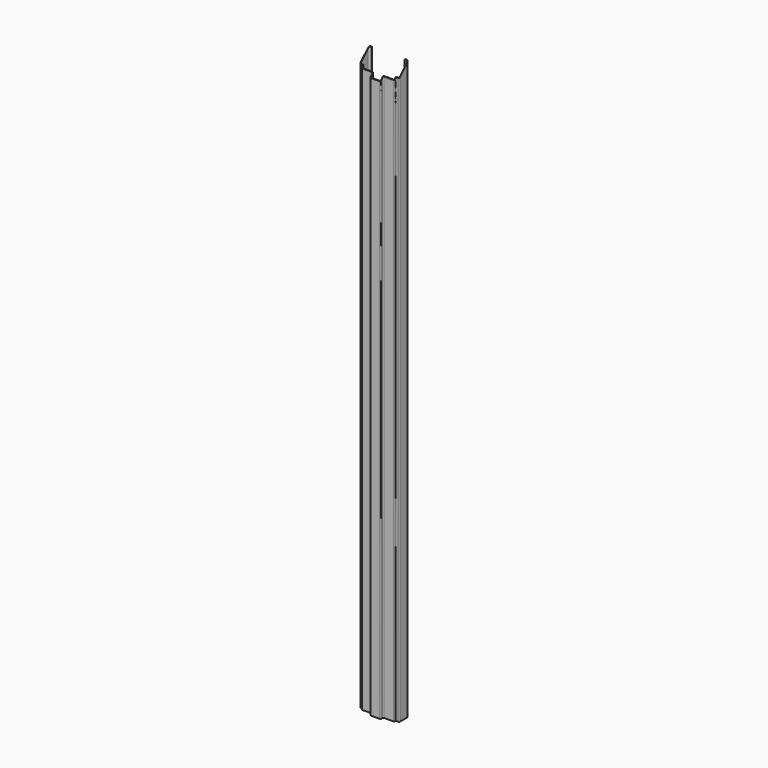
from build123d import *

# Parameters (mm, degrees)
F1_DEPTH     = 2070
F2_T1_DEPTH  = 2070
F2_T3_DEPTH  = 2070
F2_T5_DEPTH  = 2070
F2_T7_DEPTH  = 2070
F2_T9_DEPTH  = 2070
F2_T11_DEPTH = 2070
F2_T13_DEPTH = 2070
F2_T15_DEPTH = 2070
F2_T17_DEPTH = 2070
F2_T19_DEPTH = 2070
F2_T21_DEPTH = 2070
F2_T23_DEPTH = 2070
F2_T25_DEPTH = 2085
F2_T27_DEPTH = 2085
F2_T29_DEPTH = 2085
F2_T31_DEPTH = 2085
F2_T33_DEPTH = 2085
F2_T35_DEPTH = 2085
F2_T37_DEPTH = 2085
F2_T39_DEPTH = 2085
F2_T41_DEPTH = 2085
F2_T43_DEPTH = 2085
F2_T45_DEPTH = 2085
F2_T47_DEPTH = 2085
F3_R         = 5
F6_DEPTH     = 166


# Not quite as in the source:
# - a fillet or chamfer that OpenCascade refuses, or shapes differently, is made with other operations: its cross-section is extruded or revolved along the edge and cut away or added


with BuildPart() as f1:
    # F0 (on Top) → F1 (new body)
    with BuildSketch(Plane.XY):
        Polygon((-18.5, 0), (0, 0), (18.5, 0), (18.5, 12), (58.5, 12), (58.5, 19), (70.5, 19), (70.5, 60), (58.5, 60), (58.5, 57), (59.5, 57), (59.5, 59), (69.5, 59), (69.5, 20), (57.5, 20), (57.5, 13), (17.5, 13), (17.5, 1), (0, 1), (-17.5, 1), (-17.5, 13), (-57.5, 13), (-57.5, 20), (-69.5, 20), (-69.5, 59), (-59.5, 59), (-59.5, 57), (-58.5, 57), (-58.5, 60), (-70.5, 60), (-70.5, 19), (-58.5, 19), (-58.5, 12), (-18.5, 12), align=None)
    extrude(amount=F1_DEPTH)

    # F2: fillet of radius 3 on 24 edges, made by hand

    # F2_s2 → F2_t1 (join)
    with BuildSketch(Plane.XY):
        with BuildLine():
            add(Edge.make_bspline(
                [(-21.5, 12), (-18.5, 12), (-18.5, 9)],
                knots=[0, 0, 0, 1, 1, 1], degree=2, weights=[1, 1, 1]))
            Line((-18.5, 9), (-18.5, 12))
            Line((-18.5, 12), (-21.5, 12))
        make_face()
    extrude(amount=F2_T1_DEPTH)

    # F2_s4 → F2_t3 (join)
    with BuildSketch(Plane.XY):
        with BuildLine():
            add(Edge.make_bspline(
                [(-61.5, 19), (-58.5, 19), (-58.5, 16)],
                knots=[0, 0, 0, 1, 1, 1], degree=2, weights=[1, 1, 1]))
            Line((-58.5, 16), (-58.5, 19))
            Line((-58.5, 19), (-61.5, 19))
        make_face()
    extrude(amount=F2_T3_DEPTH)

    # F2_s6 → F2_t5 (join)
    with BuildSketch(Plane.XY):
        with BuildLine():
            add(Edge.make_bspline(
                [(-62.3284271247, 59), (-60.2071067812, 59), (-59.5, 57)],
                knots=[0, 0, 0, 1, 1, 1], degree=2, weights=[1, 1, 1]))
            Line((-59.5, 57), (-59.5, 59))
            Line((-59.5, 59), (-62.3284271247, 59))
        make_face()
    extrude(amount=F2_T5_DEPTH)

    # F2_s8 → F2_t7 (join)
    with BuildSketch(Plane.XY):
        with BuildLine():
            add(Edge.make_bspline(
                [(-66.5, 20), (-69.5, 20), (-69.5, 23)],
                knots=[0, 0, 0, 1, 1, 1], degree=2, weights=[1, 1, 1]))
            Line((-69.5, 23), (-69.5, 20))
            Line((-69.5, 20), (-66.5, 20))
        make_face()
    extrude(amount=F2_T7_DEPTH)

    # F2_s10 → F2_t9 (join)
    with BuildSketch(Plane.XY):
        with BuildLine():
            add(Edge.make_bspline(
                [(-54.5, 13), (-57.5, 13), (-57.5, 16)],
                knots=[0, 0, 0, 1, 1, 1], degree=2, weights=[1, 1, 1]))
            Line((-57.5, 16), (-57.5, 13))
            Line((-57.5, 13), (-54.5, 13))
        make_face()
    extrude(amount=F2_T9_DEPTH)

    # F2_s12 → F2_t11 (join)
    with BuildSketch(Plane.XY):
        with BuildLine():
            add(Edge.make_bspline(
                [(-14.5, 1), (-17.5, 1), (-17.5, 4)],
                knots=[0, 0, 0, 1, 1, 1], degree=2, weights=[1, 1, 1]))
            Line((-17.5, 4), (-17.5, 1))
            Line((-17.5, 1), (-14.5, 1))
        make_face()
    extrude(amount=F2_T11_DEPTH)

    # F2_s14 → F2_t13 (join)
    with BuildSketch(Plane.XY):
        with BuildLine():
            add(Edge.make_bspline(
                [(17.5, 4), (17.5, 1), (14.5, 1)],
                knots=[0, 0, 0, 1, 1, 1], degree=2, weights=[1, 1, 1]))
            Line((14.5, 1), (17.5, 1))
            Line((17.5, 1), (17.5, 4))
        make_face()
    extrude(amount=F2_T13_DEPTH)

    # F2_s16 → F2_t15 (join)
    with BuildSketch(Plane.XY):
        with BuildLine():
            add(Edge.make_bspline(
                [(57.5, 16), (57.5, 13), (54.5, 13)],
                knots=[0, 0, 0, 1, 1, 1], degree=2, weights=[1, 1, 1]))
            Line((54.5, 13), (57.5, 13))
            Line((57.5, 13), (57.5, 16))
        make_face()
    extrude(amount=F2_T15_DEPTH)

    # F2_s18 → F2_t17 (join)
    with BuildSketch(Plane.XY):
        with BuildLine():
            add(Edge.make_bspline(
                [(69.5, 23), (69.5, 20), (66.5, 20)],
                knots=[0, 0, 0, 1, 1, 1], degree=2, weights=[1, 1, 1]))
            Line((66.5, 20), (69.5, 20))
            Line((69.5, 20), (69.5, 23))
        make_face()
    extrude(amount=F2_T17_DEPTH)

    # F2_s20 → F2_t19 (join)
    with BuildSketch(Plane.XY):
        with BuildLine():
            add(Edge.make_bspline(
                [(59.5, 57), (60.2071067812, 59), (62.3284271247, 59)],
                knots=[0, 0, 0, 1, 1, 1], degree=2, weights=[1, 1, 1]))
            Line((62.3284271247, 59), (59.5, 59))
            Line((59.5, 59), (59.5, 57))
        make_face()
    extrude(amount=F2_T19_DEPTH)

    # F2_s22 → F2_t21 (join)
    with BuildSketch(Plane.XY):
        with BuildLine():
            add(Edge.make_bspline(
                [(58.5, 16), (58.5, 19), (61.5, 19)],
                knots=[0, 0, 0, 1, 1, 1], degree=2, weights=[1, 1, 1]))
            Line((61.5, 19), (58.5, 19))
            Line((58.5, 19), (58.5, 16))
        make_face()
    extrude(amount=F2_T21_DEPTH)

    # F2_s24 → F2_t23 (join)
    with BuildSketch(Plane.XY):
        with BuildLine():
            add(Edge.make_bspline(
                [(18.5, 9), (18.5, 12), (21.5, 12)],
                knots=[0, 0, 0, 1, 1, 1], degree=2, weights=[1, 1, 1]))
            Line((21.5, 12), (18.5, 12))
            Line((18.5, 12), (18.5, 9))
        make_face()
    extrude(amount=F2_T23_DEPTH)

    # F2_s26 → F2_t25 (cut)
    with BuildSketch(Plane.XY.offset(-7.5)):
        with BuildLine():
            add(Edge.make_bspline(
                [(-15.5, 0), (-18.5, 0), (-18.5, 3)],
                knots=[0, 0, 0, 1, 1, 1], degree=2, weights=[1, 1, 1]))
            Line((-18.5, 3), (-18.5, 0))
            Line((-18.5, 0), (-15.5, 0))
        make_face()
    extrude(amount=F2_T25_DEPTH, mode=Mode.SUBTRACT)

    # F2_s28 → F2_t27 (cut)
    with BuildSketch(Plane.XY.offset(-7.5)):
        with BuildLine():
            add(Edge.make_bspline(
                [(15.5, 0), (18.5, 0), (18.5, 3)],
                knots=[0, 0, 0, 1, 1, 1], degree=2, weights=[1, 1, 1]))
            Line((18.5, 3), (18.5, 0))
            Line((18.5, 0), (15.5, 0))
        make_face()
    extrude(amount=F2_T27_DEPTH, mode=Mode.SUBTRACT)

    # F2_s30 → F2_t29 (cut)
    with BuildSketch(Plane.XY.offset(-7.5)):
        with BuildLine():
            add(Edge.make_bspline(
                [(-55.5, 12), (-58.5, 12), (-58.5, 15)],
                knots=[0, 0, 0, 1, 1, 1], degree=2, weights=[1, 1, 1]))
            Line((-58.5, 15), (-58.5, 12))
            Line((-58.5, 12), (-55.5, 12))
        make_face()
    extrude(amount=F2_T29_DEPTH, mode=Mode.SUBTRACT)

    # F2_s32 → F2_t31 (cut)
    with BuildSketch(Plane.XY.offset(-7.5)):
        with BuildLine():
            add(Edge.make_bspline(
                [(-67.5, 19), (-70.5, 19), (-70.5, 22)],
                knots=[0, 0, 0, 1, 1, 1], degree=2, weights=[1, 1, 1]))
            Line((-70.5, 22), (-70.5, 19))
            Line((-70.5, 19), (-67.5, 19))
        make_face()
    extrude(amount=F2_T31_DEPTH, mode=Mode.SUBTRACT)

    # F2_s34 → F2_t33 (cut)
    with BuildSketch(Plane.XY.offset(-7.5)):
        with BuildLine():
            add(Edge.make_bspline(
                [(-61.5, 60), (-58.5, 60), (-58.5, 57)],
                knots=[0, 0, 0, 1, 1, 1], degree=2, weights=[1, 1, 1]))
            Line((-58.5, 57), (-58.5, 60))
            Line((-58.5, 60), (-61.5, 60))
        make_face()
    extrude(amount=F2_T33_DEPTH, mode=Mode.SUBTRACT)

    # F2_s36 → F2_t35 (cut)
    with BuildSketch(Plane.XY.offset(-7.5)):
        with BuildLine():
            add(Edge.make_bspline(
                [(-60.5, 20), (-57.5, 20), (-57.5, 17)],
                knots=[0, 0, 0, 1, 1, 1], degree=2, weights=[1, 1, 1]))
            Line((-57.5, 17), (-57.5, 20))
            Line((-57.5, 20), (-60.5, 20))
        make_face()
    extrude(amount=F2_T35_DEPTH, mode=Mode.SUBTRACT)

    # F2_s38 → F2_t37 (cut)
    with BuildSketch(Plane.XY.offset(-7.5)):
        with BuildLine():
            add(Edge.make_bspline(
                [(-20.5, 13), (-17.5, 13), (-17.5, 10)],
                knots=[0, 0, 0, 1, 1, 1], degree=2, weights=[1, 1, 1]))
            Line((-17.5, 10), (-17.5, 13))
            Line((-17.5, 13), (-20.5, 13))
        make_face()
    extrude(amount=F2_T37_DEPTH, mode=Mode.SUBTRACT)

    # F2_s40 → F2_t39 (cut)
    with BuildSketch(Plane.XY.offset(-7.5)):
        with BuildLine():
            add(Edge.make_bspline(
                [(17.5, 10), (17.5, 13), (20.5, 13)],
                knots=[0, 0, 0, 1, 1, 1], degree=2, weights=[1, 1, 1]))
            Line((20.5, 13), (17.5, 13))
            Line((17.5, 13), (17.5, 10))
        make_face()
    extrude(amount=F2_T39_DEPTH, mode=Mode.SUBTRACT)

    # F2_s42 → F2_t41 (cut)
    with BuildSketch(Plane.XY.offset(-7.5)):
        with BuildLine():
            add(Edge.make_bspline(
                [(57.5, 17), (57.5, 20), (60.5, 20)],
                knots=[0, 0, 0, 1, 1, 1], degree=2, weights=[1, 1, 1]))
            Line((60.5, 20), (57.5, 20))
            Line((57.5, 20), (57.5, 17))
        make_face()
    extrude(amount=F2_T41_DEPTH, mode=Mode.SUBTRACT)

    # F2_s44 → F2_t43 (cut)
    with BuildSketch(Plane.XY.offset(-7.5)):
        with BuildLine():
            add(Edge.make_bspline(
                [(58.5, 57), (58.5, 60), (61.5, 60)],
                knots=[0, 0, 0, 1, 1, 1], degree=2, weights=[1, 1, 1]))
            Line((61.5, 60), (58.5, 60))
            Line((58.5, 60), (58.5, 57))
        make_face()
    extrude(amount=F2_T43_DEPTH, mode=Mode.SUBTRACT)

    # F2_s46 → F2_t45 (cut)
    with BuildSketch(Plane.XY.offset(-7.5)):
        with BuildLine():
            add(Edge.make_bspline(
                [(70.5, 22), (70.5, 19), (67.5, 19)],
                knots=[0, 0, 0, 1, 1, 1], degree=2, weights=[1, 1, 1]))
            Line((67.5, 19), (70.5, 19))
            Line((70.5, 19), (70.5, 22))
        make_face()
    extrude(amount=F2_T45_DEPTH, mode=Mode.SUBTRACT)

    # F2_s48 → F2_t47 (cut)
    with BuildSketch(Plane.XY.offset(-7.5)):
        with BuildLine():
            add(Edge.make_bspline(
                [(58.5, 15), (58.5, 12), (55.5, 12)],
                knots=[0, 0, 0, 1, 1, 1], degree=2, weights=[1, 1, 1]))
            Line((55.5, 12), (58.5, 12))
            Line((58.5, 12), (58.5, 15))
        make_face()
    extrude(amount=F2_T47_DEPTH, mode=Mode.SUBTRACT)

    # F3
    f3_edges = [f1.edges().sort_by_distance(p)[0] for p in [
        (-70.5, 60, 1035),
        (-69.5, 59, 1035),
        (70.5, 60, 1035),
        (69.5, 59, 1035),
    ]]
    fillet(f3_edges, radius=F3_R)

    # F5 (on offset) → F6 (cut)
    with BuildSketch(Plane.YZ.offset(70.5)):
        Polygon((-1.5182899632, 2008.4817100368), (60, 2070), (-11.1059369519, 2070), align=None)
    extrude(amount=-F6_DEPTH, mode=Mode.SUBTRACT)


solid = f1.part
